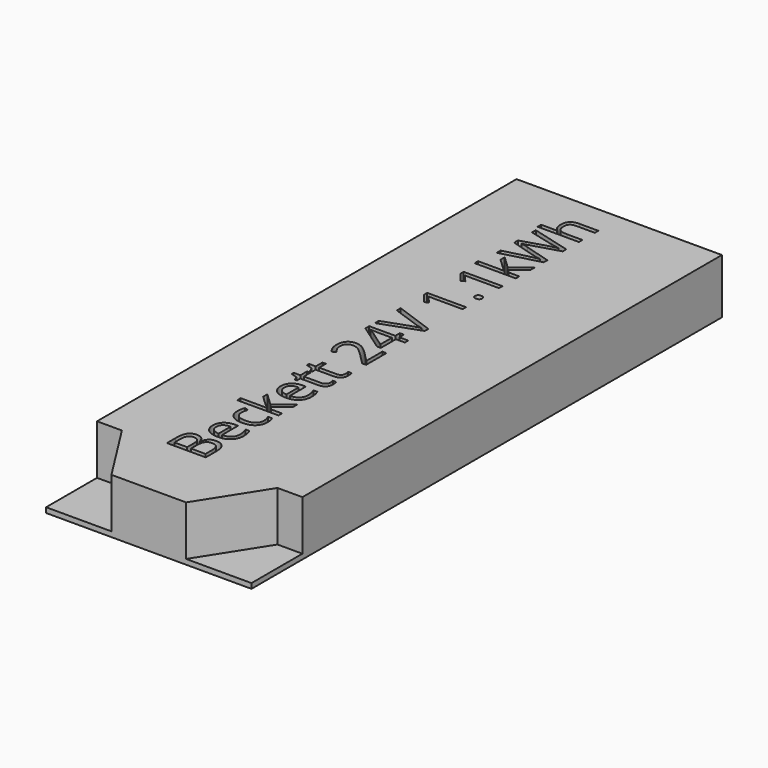
from build123d import *

# Parameters (mm, degrees)
F0_W         = 209.55
F0_H         = 600
F1_DEPTH     = 56
F3_DEPTH     = 50.8
F4_TEXT_SIZE = 55.4485629609
F5_DEPTH     = 25.4


# Not quite as in the source:
# - Text() gives the source's letters only with a copy of the font that has no kerning and outlines rounded to 1/6400 em; it was checked with that copy


with BuildPart() as f1:
    # F0 (on Top) → F1 (new body)
    with BuildSketch(Plane.XY):
        with Locations((104.775, 300)):
            Rectangle(F0_W, F0_H)
    extrude(amount=F1_DEPTH)

    # F2 (on face) → F3 (cut)
    with BuildSketch(Plane.XY.offset(56)):
        Polygon((142.875, 0), (209.55, 0), (209.55, 64.9413913488), (184.15, 64.9413913488), align=None)
        Polygon((0, 64.9413913488), (0, 0), (66.675, 0), (25.4, 64.9413913488), align=None)
    extrude(amount=-F3_DEPTH, mode=Mode.SUBTRACT)

    # F4 (on face) → F5 (cut)
    with BuildSketch(Plane.XY.offset(56)):
        with Locations(Location((106.5979653319, 64.9413913488), (0, 0, 90))):
            Text('Beckett 24V 1.1kWh', F4_TEXT_SIZE, font='Open Sans', text_align=(TextAlign.LEFT, TextAlign.BOTTOM))
    extrude(amount=-F5_DEPTH, mode=Mode.SUBTRACT)


solid = f1.part
